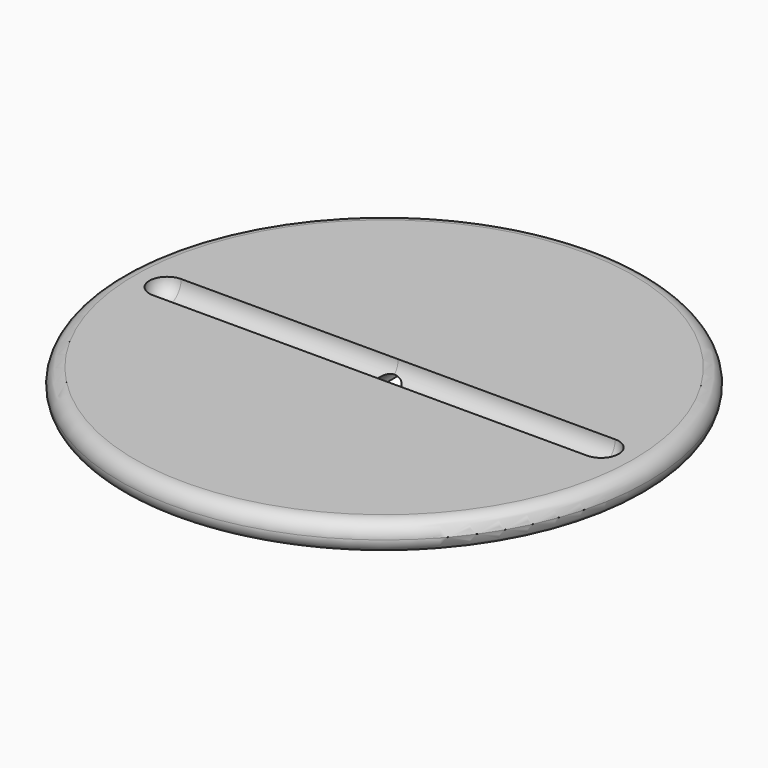
from build123d import *

# Parameters (mm, degrees)
F0_R          = 90
F1_DEPTH      = 10
F2_R          = 4.99999
F3_R          = 6
F4_DEPTH      = 80
F4_DEPTH_BACK = 80
F5_R          = 6
F6_DEPTH      = 80
F6_DEPTH_BACK = 80
F7_R          = 5.99999
F8_R          = 5.99999


# Not quite as in the source:
# - a fillet or chamfer is up to 0.001 mm smaller than in the source, because OpenCascade refuses the exact size


with BuildPart() as f1:
    # F0 (on Top) → F1 (new body)
    with BuildSketch(Plane.XY):
        Circle(F0_R)
    extrude(amount=F1_DEPTH)

    # F2 (radius 5 in the source; OpenCascade refuses exactly that, so slightly less here)
    f2_edges = [f1.edges().sort_by_distance(p)[0] for p in [
        (-90, 0, 10),
        (-90, 0, 0),
    ]]
    fillet(f2_edges, radius=F2_R)

    # F3 (on Front) → F4 (cut, two sides)
    with BuildSketch(Plane.XZ) as f4_sk:
        Circle(F3_R)
    extrude(amount=F4_DEPTH, mode=Mode.SUBTRACT)
    extrude(f4_sk.sketch, amount=-F4_DEPTH_BACK, mode=Mode.SUBTRACT)

    # F5 (on Right) → F6 (cut, two sides)
    with BuildSketch(Plane.YZ) as f6_sk:
        with Locations((0, 10)):
            Circle(F5_R)
    extrude(amount=-F6_DEPTH, mode=Mode.SUBTRACT)
    extrude(f6_sk.sketch, amount=F6_DEPTH_BACK, mode=Mode.SUBTRACT)

    # F7 (radius 6 in the source; OpenCascade refuses exactly that, so slightly less here)
    f7_edges = [f1.edges().sort_by_distance(p)[0] for p in [
        (80, 0, 4),
        (-80, 0, 4),
    ]]
    fillet(f7_edges, radius=F7_R)

    # F8 (radius 6 in the source; OpenCascade refuses exactly that, so slightly less here)
    f8_edges = [f1.edges().sort_by_distance(p)[0] for p in [
        (0, -80, 6),
        (0, 80, 6),
    ]]
    fillet(f8_edges, radius=F8_R)


solid = f1.part
